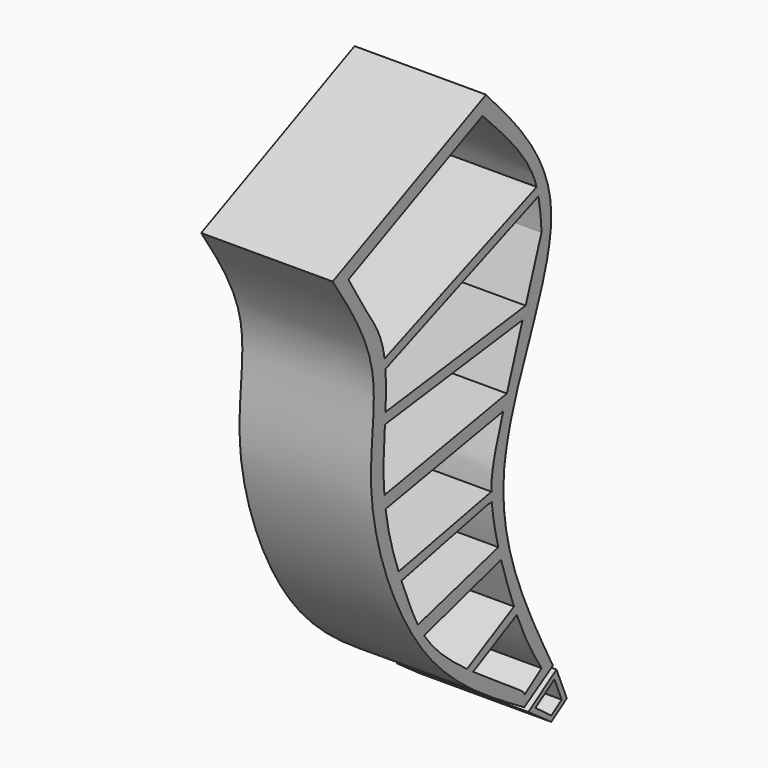
from build123d import *

# Parameters (mm, degrees)
F1_DEPTH  = 25
F2_DEPTH  = 25
F3_DEPTH  = 25
F4_DEPTH  = 25
F5_DEPTH  = 25
F6_DEPTH  = 25
F7_DEPTH  = 25
F10_DEPTH = 1
F11_DEPTH = 1


with BuildPart() as f1:
    # F0 (on Right) → F1 (new body)
    with BuildSketch(Plane.YZ):
        with BuildLine():
            Line((76.8012625446, 52.4432235212), (40.3474546597, 35.9775048702))
            add(Edge.make_bspline(
                [(40.3474546597, 35.9775048702), (44.5158897869, 29.6814892591), (52.7818571842, 17.1992282489), (46.5552937226, -3.8418948455), (59.8918941993, -37.9753033909), (77.3855119754, -48.6559954876), (85.8946596675, -53.8051620452)],
                knots=[0, 0, 0, 0, 0.225066194, 0.4463115245, 0.7316938963, 1, 1, 1, 1], degree=3))
            Line((85.8946596675, -53.8051620452), (92.699803412, -49.599211663))
            add(Edge.make_bspline(
                [(76.8012625446, 52.4432235212), (84.5131378217, 44.1641811003), (100.9174434445, 26.5534266137), (73.0582859494, -12.006269763), (86.1284394595, -37.021929702), (92.699803412, -49.599211663)],
                knots=[0, 0, 0, 0, 0.3061020156, 0.6511245107, 1, 1, 1, 1], degree=3))
        make_face()
        with BuildLine():
            add(Edge.make_bspline(
                [(44.102743268, 34.7667783499), (45.5869866773, 32.2564890577), (48.3654293439, 27.5573155976), (51.5365048206, 23.133247426), (52.4618114074, 19.5054126847), (52.6898807242, 18.0451917615)],
                knots=[0, 0, 0, 0, 0.1013554355, 0.1897091451, 0.2415289385, 0.2415289385, 0.2415289385, 0.2415289385], degree=3))
            Line((44.102743268, 34.7667783499), (75.9686642859, 49.2430719943))
            add(Edge.make_bspline(
                [(75.9686642859, 49.2430719943), (80.7651980081, 44.3752599295), (86.4678121426, 38.5879027477), (88.5720183844, 32.9802603832), (88.8379309187, 32.0926870872)],
                knots=[0, 0, 0, 0, 0.5664602164, 0.6734663454, 0.6734663454, 0.6734663454, 0.6734663454], degree=3))
            add(Edge.make_bspline(
                [(88.8379309187, 32.0926870872), (89.0099371396, 31.5185579706), (89.1533143996, 30.9458586664), (89.2741313424, 30.3742860892)],
                knots=[0.6734663454, 0.6734663454, 0.6734663454, 0.6734663454, 0.7426835409, 0.7426835409, 0.7426835409, 0.7426835409], degree=3))
            add(Edge.make_bspline(
                [(89.2741313424, 30.3742860892), (89.7232710063, 28.2494523594), (89.8606277376, 26.140189964), (89.9979844689, 24.0309275687)],
                knots=[0.7426835409, 0.7426835409, 0.7426835409, 0.7426835409, 1, 1, 1, 1], degree=3))
            add(Edge.make_bspline(
                [(89.9979844689, 24.0309275687), (88.756802073, 20.5110691156), (87.5156196771, 16.9912106625), (86.221231401, 13.2950814443)],
                knots=[0, 0, 0, 0, 0.1371374041, 0.1371374041, 0.1371374041, 0.1371374041], degree=3))
            add(Edge.make_bspline(
                [(86.221231401, 13.2950814443), (85.977143483, 12.5980877352), (85.7311635566, 11.8948258136), (85.4829348383, 11.1841136579)],
                knots=[0.1371374041, 0.1371374041, 0.1371374041, 0.1371374041, 0.162997947, 0.162997947, 0.162997947, 0.162997947], degree=3))
            add(Edge.make_bspline(
                [(85.4829348383, 11.1841136579), (85.267818915, 10.568207881), (84.035080256, 7.0343916925), (82.7402342637, 3.2948142782), (81.7634153644, 0.4019179056)],
                knots=[0.162997947, 0.162997947, 0.162997947, 0.162997947, 0.1854087888, 0.2904246225, 0.2904246225, 0.2904246225, 0.2904246225], degree=3))
            add(Edge.make_bspline(
                [(81.7634153644, 0.4019179056), (81.4591421255, -0.4992019947), (81.1636304992, -1.3819842427), (80.8808845893, -2.2364929875)],
                knots=[0.2904246225, 0.2904246225, 0.2904246225, 0.2904246225, 0.3231364259, 0.3231364259, 0.3231364259, 0.3231364259], degree=3))
            add(Edge.make_bspline(
                [(80.8808845893, -2.2364929875), (80.4400262019, -3.5688459381), (78.9176886377, -8.2626995613), (78.0330144779, -11.4884184754), (78.0771449208, -14.5385963842)],
                knots=[0.3231364259, 0.3231364259, 0.3231364259, 0.3231364259, 0.3741407815, 0.5125981189, 0.5125981189, 0.5125981189, 0.5125981189], degree=3))
            add(Edge.make_bspline(
                [(78.0771449208, -14.5385963842), (78.0854311956, -15.1113214854), (78.1180673371, -15.708474008), (78.1726109732, -16.3263524444)],
                knots=[0.5125981189, 0.5125981189, 0.5125981189, 0.5125981189, 0.5385959443, 0.5385959443, 0.5385959443, 0.5385959443], degree=3))
            add(Edge.make_bspline(
                [(78.1726109732, -16.3263524444), (78.3908448139, -18.7985379066), (78.9597891259, -21.6025182715), (79.7230046196, -24.5012038636)],
                knots=[0.5385959443, 0.5385959443, 0.5385959443, 0.5385959443, 0.6426155089, 0.6426155089, 0.6426155089, 0.6426155089], degree=3))
            add(Edge.make_bspline(
                [(79.7230046196, -24.5012038636), (79.9288007209, -25.2828156082), (80.1487218174, -26.0713131446), (80.3797008955, -26.8620482969)],
                knots=[0.6426155089, 0.6426155089, 0.6426155089, 0.6426155089, 0.6706637089, 0.6706637089, 0.6706637089, 0.6706637089], degree=3))
            add(Edge.make_bspline(
                [(80.3797008955, -26.8620482969), (80.5346897961, -27.3926382232), (81.4658723686, -30.4871004032), (82.53436506, -33.5681161087), (83.4502053618, -35.9443889597)],
                knots=[0.6706637089, 0.6706637089, 0.6706637089, 0.6706637089, 0.6894842867, 0.7802194818, 0.7802194818, 0.7802194818, 0.7802194818], degree=3))
            add(Edge.make_bspline(
                [(83.4502053618, -35.9443889597), (83.6683649907, -36.5104339378), (83.8882781867, -37.0665231191), (84.109089606, -37.61040963)],
                knots=[0.7802194818, 0.7802194818, 0.7802194818, 0.7802194818, 0.8018332462, 0.8018332462, 0.8018332462, 0.8018332462], degree=3))
            add(Edge.make_bspline(
                [(84.109089606, -37.61040963), (84.8138660141, -39.3463632453), (86.8646706616, -43.9759146648), (88.7614879392, -46.9768327841), (89.9979844689, -48.933070153)],
                knots=[0.8018332462, 0.8018332462, 0.8018332462, 0.8018332462, 0.8708191315, 1, 1, 1, 1], degree=3))
            add(Edge.make_bspline(
                [(89.9979844689, -48.933070153), (88.6734475692, -49.8509593308), (87.3239142246, -50.7842976763), (85.9993773248, -51.7021868541)],
                knots=[0, 0, 0, 0, 4.8638324804, 4.8638324804, 4.8638324804, 4.8638324804], degree=3))
            add(Edge.make_bspline(
                [(73.7536014428, -42.9259891452), (79.2616839922, -46.8631805496), (86.037278468, -51.0030413418), (85.9922818168, -51.6108465033), (85.9993773248, -51.7021868541)],
                knots=[0.8608913016, 0.8608913016, 0.8608913016, 0.8608913016, 0.9773228143, 1, 1, 1, 1], degree=3))
            add(Edge.make_bspline(
                [(72.2871573894, -41.8626360836), (72.7723382988, -42.2198965256), (73.2623216333, -42.5748210889), (73.7536014428, -42.9259891452)],
                knots=[0.8505064806, 0.8505064806, 0.8505064806, 0.8505064806, 0.8608913016, 0.8608913016, 0.8608913016, 0.8608913016], degree=3))
            add(Edge.make_bspline(
                [(62.0953731802, -32.1328573769), (63.2607762114, -33.8249216397), (65.9221012078, -36.948023318), (70.276587401, -40.3821633179), (72.2871573894, -41.8626360836)],
                knots=[0.7533164578, 0.7533164578, 0.7533164578, 0.7533164578, 0.807472204, 0.8505064806, 0.8505064806, 0.8505064806, 0.8505064806], degree=3))
            add(Edge.make_bspline(
                [(60.6140407616, -29.7249532229), (61.0500389658, -30.5200602261), (61.5361490607, -31.3209123912), (62.0953731802, -32.1328573769)],
                knots=[0.7273295685, 0.7273295685, 0.7273295685, 0.7273295685, 0.7533164578, 0.7533164578, 0.7533164578, 0.7533164578], degree=3))
            add(Edge.make_bspline(
                [(56.7143509479, -20.7657126474), (57.2022867526, -22.0176289299), (58.4314466262, -25.0352506359), (59.6503652252, -27.9675488107), (60.6140407616, -29.7249532229)],
                knots=[0.629936332, 0.629936332, 0.629936332, 0.629936332, 0.6698914204, 0.7273295685, 0.7273295685, 0.7273295685, 0.7273295685], degree=3))
            add(Edge.make_bspline(
                [(56.023799175, -18.9501089583), (56.2488718487, -19.5585059667), (56.479724527, -20.1637223163), (56.7143509479, -20.7657126474)],
                knots=[0.6107237239, 0.6107237239, 0.6107237239, 0.6107237239, 0.629936332, 0.629936332, 0.629936332, 0.629936332], degree=3))
            add(Edge.make_bspline(
                [(52.9298675724, -7.2175439477), (53.1930874664, -9.0898648938), (53.9905101976, -13.0627263871), (55.2720652308, -16.9180866991), (56.023799175, -18.9501089583)],
                knots=[0.4910644354, 0.4910644354, 0.4910644354, 0.4910644354, 0.5465543628, 0.6107237239, 0.6107237239, 0.6107237239, 0.6107237239], degree=3))
            add(Edge.make_bspline(
                [(52.6497218639, -4.78632948), (52.7232859651, -5.6025209503), (52.816732962, -6.4128011999), (52.9298675724, -7.2175439477)],
                knots=[0.4672142955, 0.4672142955, 0.4672142955, 0.4672142955, 0.4910644354, 0.4910644354, 0.4910644354, 0.4910644354], degree=3))
            add(Edge.make_bspline(
                [(52.7753754315, 6.992655232), (52.6218918281, 4.68010238), (52.3429405378, 0.660525646), (52.5079813052, -3.2137222818), (52.6497218639, -4.78632948)],
                knots=[0.3555619538, 0.3555619538, 0.3555619538, 0.3555619538, 0.4212607378, 0.4672142955, 0.4672142955, 0.4672142955, 0.4672142955], degree=3))
            add(Edge.make_bspline(
                [(52.9043617104, 9.0255401907), (52.8651208941, 8.3542760315), (52.8207131366, 7.6757629835), (52.7753754315, 6.992655232)],
                knots=[0.3361551115, 0.3361551115, 0.3361551115, 0.3361551115, 0.3555619538, 0.3555619538, 0.3555619538, 0.3555619538], degree=3))
            add(Edge.make_bspline(
                [(52.9090998165, 16.242469639), (52.9936284832, 15.2983602445), (53.0966265832, 12.9902209855), (52.9901220017, 10.4925792381), (52.9043617104, 9.0255401907)],
                knots=[0.2622006915, 0.2622006915, 0.2622006915, 0.2622006915, 0.2937417112, 0.3361551115, 0.3361551115, 0.3361551115, 0.3361551115], degree=3))
            add(Edge.make_bspline(
                [(52.6898807242, 18.0451917615), (52.7808612605, 17.4626860367), (52.8537003481, 16.8612320142), (52.9090998165, 16.242469639)],
                knots=[0.2415289385, 0.2415289385, 0.2415289385, 0.2415289385, 0.2622006915, 0.2622006915, 0.2622006915, 0.2622006915], degree=3))
        make_face(mode=Mode.SUBTRACT)
    extrude(amount=F1_DEPTH)

    # F0 (on Right) → F2 (join)
    with BuildSketch(Plane.YZ):
        with BuildLine():
            Line((88.8379309186, 32.0926870872), (52.6898807242, 18.0451917615))
            add(Edge.make_bspline(
                [(52.6898807242, 18.0451917615), (52.7808612605, 17.4626860367), (52.8537003481, 16.8612320142), (52.9090998165, 16.242469639)],
                knots=[0.2415289385, 0.2415289385, 0.2415289385, 0.2415289385, 0.2622006915, 0.2622006915, 0.2622006915, 0.2622006915], degree=3))
            Line((52.9090998165, 16.242469639), (89.2741313424, 30.3742860892))
            add(Edge.make_bspline(
                [(88.8379309187, 32.0926870872), (89.0099371396, 31.5185579706), (89.1533143996, 30.9458586664), (89.2741313424, 30.3742860892)],
                knots=[0.6734663454, 0.6734663454, 0.6734663454, 0.6734663454, 0.7426835409, 0.7426835409, 0.7426835409, 0.7426835409], degree=3))
        make_face()
    extrude(amount=F2_DEPTH)

    # F0 (on Right) → F3 (join)
    with BuildSketch(Plane.YZ):
        with BuildLine():
            Line((86.221231401, 13.2950814443), (52.9043617104, 9.0255401907))
            add(Edge.make_bspline(
                [(52.9043617104, 9.0255401907), (52.8651208941, 8.3542760315), (52.8207131366, 7.6757629835), (52.7753754315, 6.992655232)],
                knots=[0.3361551115, 0.3361551115, 0.3361551115, 0.3361551115, 0.3555619538, 0.3555619538, 0.3555619538, 0.3555619538], degree=3))
            Line((52.7753754315, 6.992655232), (85.4829348383, 11.1841136579))
            add(Edge.make_bspline(
                [(86.221231401, 13.2950814443), (85.977143483, 12.5980877352), (85.7311635566, 11.8948258136), (85.4829348383, 11.1841136579)],
                knots=[0.1371374041, 0.1371374041, 0.1371374041, 0.1371374041, 0.162997947, 0.162997947, 0.162997947, 0.162997947], degree=3))
        make_face()
    extrude(amount=F3_DEPTH)

    # F0 (on Right) → F4 (join)
    with BuildSketch(Plane.YZ):
        with BuildLine():
            Line((81.7634153644, 0.4019179056), (52.6497218639, -4.78632948))
            add(Edge.make_bspline(
                [(52.6497218639, -4.78632948), (52.7232859651, -5.6025209503), (52.816732962, -6.4128011999), (52.9298675724, -7.2175439477)],
                knots=[0.4672142955, 0.4672142955, 0.4672142955, 0.4672142955, 0.4910644354, 0.4910644354, 0.4910644354, 0.4910644354], degree=3))
            Line((52.9298675724, -7.2175439477), (80.8808845893, -2.2364929875))
            add(Edge.make_bspline(
                [(81.7634153644, 0.4019179056), (81.4591421255, -0.4992019947), (81.1636304992, -1.3819842427), (80.8808845893, -2.2364929875)],
                knots=[0.2904246225, 0.2904246225, 0.2904246225, 0.2904246225, 0.3231364259, 0.3231364259, 0.3231364259, 0.3231364259], degree=3))
        make_face()
    extrude(amount=F4_DEPTH)

    # F0 (on Right) → F5 (join)
    with BuildSketch(Plane.YZ):
        with BuildLine():
            Line((78.0771449208, -14.5385963842), (56.023799175, -18.9501089583))
            add(Edge.make_bspline(
                [(56.023799175, -18.9501089583), (56.2488718487, -19.5585059667), (56.479724527, -20.1637223163), (56.7143509479, -20.7657126474)],
                knots=[0.6107237239, 0.6107237239, 0.6107237239, 0.6107237239, 0.629936332, 0.629936332, 0.629936332, 0.629936332], degree=3))
            Line((56.7143509479, -20.7657126474), (77.2671707729, -16.3263524444))
            Line((77.2671707729, -16.3263524444), (78.1726109732, -16.3263524444))
            add(Edge.make_bspline(
                [(78.0771449208, -14.5385963842), (78.0854311956, -15.1113214854), (78.1180673371, -15.708474008), (78.1726109732, -16.3263524444)],
                knots=[0.5125981189, 0.5125981189, 0.5125981189, 0.5125981189, 0.5385959443, 0.5385959443, 0.5385959443, 0.5385959443], degree=3))
        make_face()
    extrude(amount=F5_DEPTH)

    # F0 (on Right) → F6 (join)
    with BuildSketch(Plane.YZ):
        with BuildLine():
            Line((79.7230046196, -24.5012038636), (60.6140407616, -29.7249532229))
            add(Edge.make_bspline(
                [(60.6140407616, -29.7249532229), (61.0500389658, -30.5200602261), (61.5361490607, -31.3209123912), (62.0953731802, -32.1328573769)],
                knots=[0.7273295685, 0.7273295685, 0.7273295685, 0.7273295685, 0.7533164578, 0.7533164578, 0.7533164578, 0.7533164578], degree=3))
            Line((62.0953731802, -32.1328573769), (80.3797008955, -26.8620482969))
            add(Edge.make_bspline(
                [(79.7230046196, -24.5012038636), (79.9288007209, -25.2828156082), (80.1487218174, -26.0713131446), (80.3797008955, -26.8620482969)],
                knots=[0.6426155089, 0.6426155089, 0.6426155089, 0.6426155089, 0.6706637089, 0.6706637089, 0.6706637089, 0.6706637089], degree=3))
        make_face()
    extrude(amount=F6_DEPTH)

    # F0 (on Right) → F7 (join)
    with BuildSketch(Plane.YZ):
        with BuildLine():
            Line((83.4502053618, -35.9443889597), (72.2871573894, -41.8626360836))
            add(Edge.make_bspline(
                [(72.2871573894, -41.8626360836), (72.7723382988, -42.2198965256), (73.2623216333, -42.5748210889), (73.7536014428, -42.9259891452)],
                knots=[0.8505064806, 0.8505064806, 0.8505064806, 0.8505064806, 0.8608913016, 0.8608913016, 0.8608913016, 0.8608913016], degree=3))
            Line((73.7536014428, -42.9259891452), (84.109089606, -37.61040963))
            add(Edge.make_bspline(
                [(83.4502053618, -35.9443889597), (83.6683649907, -36.5104339378), (83.8882781867, -37.0665231191), (84.109089606, -37.61040963)],
                knots=[0.7802194818, 0.7802194818, 0.7802194818, 0.7802194818, 0.8018332462, 0.8018332462, 0.8018332462, 0.8018332462], degree=3))
        make_face()
    extrude(amount=F7_DEPTH)


with BuildPart() as f1b:
    # F0 (on Right) → F1, piece 2 (new body)
    with BuildSketch(Plane.YZ):
        Polygon((93.5478610859, -50.5871062748), (86.8721157312, -54.9955554307), (92.3091694713, -58.8661059737), (96.0069314157, -56.4242220108), align=None)
        Polygon((92.3091694713, -57.8015310683), (88.5542035103, -54.9955554307), (93.0576155611, -52.0216458522), (94.7997059314, -56.156860283), align=None, mode=Mode.SUBTRACT)
    extrude(amount=F1_DEPTH)


with BuildPart() as f10:
    # F9 (on offset) → F10 (new body)
    with BuildSketch(Plane(origin=(0, 0, 0), x_dir=(0, -1, 0), z_dir=(-1, 0, 0))):
        with BuildLine():
            add(Edge.make_bspline(
                [(-75.9686642859, 49.2430719943), (-65.3466906133, 44.4176407795), (-54.7247169407, 39.5922095647), (-44.102743268, 34.7667783499)],
                knots=[0, 0, 0, 0, 35, 35, 35, 35], degree=3))
            add(Edge.make_bspline(
                [(-75.9686642859, 49.2430719943), (-78.66129457, 46.6755219245), (-83.9903281299, 41.5940368911), (-87.233469527, 35.2374474134), (-88.837930919, 32.0926870862)],
                knots=[0, 0, 0, 0, 0.5052755352, 1, 1, 1, 1], degree=3))
            add(Edge.make_bspline(
                [(-88.837930919, 32.0926870862), (-76.788580854, 27.4101886451), (-64.739230789, 22.7276902041), (-52.689880724, 18.0451917631)],
                knots=[0, 0, 0, 0, 38.7816149451, 38.7816149451, 38.7816149451, 38.7816149451], degree=3))
            add(Edge.make_bspline(
                [(-44.102743268, 34.7667783499), (-45.8580037651, 31.8560220837), (-48.8950957621, 26.8196078013), (-51.8328315201, 22.5455398579), (-52.4106929353, 19.5112090299), (-52.689880724, 18.0451917631)],
                knots=[0, 0, 0, 0, 0.4144400443, 0.7170897725, 1, 1, 1, 1], degree=3))
        make_face()
    extrude(amount=-F10_DEPTH)


with BuildPart() as f10b:
    # F9 (on offset) → F10, piece 2 (new body)
    with BuildSketch(Plane(origin=(0, 0, 0), x_dir=(0, -1, 0), z_dir=(-1, 0, 0))):
        with BuildLine():
            add(Edge.make_bspline(
                [(-89.2741313426, 30.3742860884), (-77.1524541671, 25.663680606), (-65.0307769917, 20.9530751235), (-52.9090998163, 16.2424696411)],
                knots=[0, 0, 0, 0, 39.0144044426, 39.0144044426, 39.0144044426, 39.0144044426], degree=3))
            add(Edge.make_bspline(
                [(-89.2741313426, 30.3742860884), (-89.8685955616, 28.5150743963), (-91.2921272563, 24.062919521), (-88.0875709088, 17.2581763669), (-86.2212314015, 13.2950814457)],
                knots=[0, 0, 0, 0, 0.4175981618, 1, 1, 1, 1], degree=3))
            add(Edge.make_bspline(
                [(-52.9043617106, 9.0255401932), (-64.0099849409, 10.4487206107), (-75.1156081712, 11.8719010282), (-86.2212314015, 13.2950814457)],
                knots=[0, 0, 0, 0, 33.5893255143, 33.5893255143, 33.5893255143, 33.5893255143], degree=3))
            add(Edge.make_bspline(
                [(-52.9090998163, 16.2424696411), (-52.9075204477, 13.8368264918), (-52.9059410791, 11.4311833425), (-52.9043617106, 9.0255401932)],
                knots=[0, 0, 0, 0, 7.2169310032, 7.2169310032, 7.2169310032, 7.2169310032], degree=3))
        make_face()
    extrude(amount=-F10_DEPTH)


with BuildPart() as f10c:
    # F9 (on offset) → F10, piece 3 (new body)
    with BuildSketch(Plane(origin=(0, 0, 0), x_dir=(0, -1, 0), z_dir=(-1, 0, 0))):
        with BuildLine():
            add(Edge.make_bspline(
                [(-85.4829348402, 11.1841136634), (-74.5804150374, 9.7869608546), (-63.6778952346, 8.3898080457), (-52.7753754318, 6.9926552369)],
                knots=[0, 0, 0, 0, 32.9750324669, 32.9750324669, 32.9750324669, 32.9750324669], degree=3))
            add(Edge.make_bspline(
                [(-85.4829348402, 11.1841136634), (-84.2430950149, 7.5900484108), (-83.0032551897, 3.9959831582), (-81.7634153644, 0.4019179056)],
                knots=[0, 0, 0, 0, 11.4057253382, 11.4057253382, 11.4057253382, 11.4057253382], degree=3))
            add(Edge.make_bspline(
                [(-52.6497218631, -4.7863294703), (-62.3542863635, -3.0569136783), (-72.058850864, -1.3274978864), (-81.7634153644, 0.4019179056)],
                knots=[0, 0, 0, 0, 29.5723698767, 29.5723698767, 29.5723698767, 29.5723698767], degree=3))
            add(Edge.make_bspline(
                [(-52.7753754318, 6.9926552369), (-52.629764464, 5.0302460442), (-52.3385765641, 1.1058863612), (-52.5460148456, -2.8224105807), (-52.6497218631, -4.7863294703)],
                knots=[0, 0, 0, 0, 0.500058443, 1, 1, 1, 1], degree=3))
        make_face()
    extrude(amount=-F10_DEPTH)


with BuildPart() as f10d:
    # F9 (on offset) → F10, piece 4 (new body)
    with BuildSketch(Plane(origin=(0, 0, 0), x_dir=(0, -1, 0), z_dir=(-1, 0, 0))):
        with BuildLine():
            add(Edge.make_bspline(
                [(-80.8808845893, -2.2364929876), (-71.5638789166, -3.8968433045), (-62.2468732438, -5.5571936213), (-52.9298675711, -7.2175439382)],
                knots=[0, 0, 0, 0, 28.3913758196, 28.3913758196, 28.3913758196, 28.3913758196], degree=3))
            add(Edge.make_bspline(
                [(-80.8808845893, -2.2364929876), (-80.1631109469, -4.2347182609), (-78.7288687651, -8.2275378818), (-78.2942557626, -12.4361863007), (-78.0771449208, -14.5385963842)],
                knots=[0, 0, 0, 0, 0.5004567325, 1, 1, 1, 1], degree=3))
            Line((-78.0771449208, -14.5385963842), (-56.0237991752, -19.1139187664))
            add(Edge.make_bspline(
                [(-52.9298675711, -7.2175439382), (-53.2836007921, -9.2084246591), (-53.9956375963, -13.2158988545), (-55.3448600225, -17.1395203588), (-56.0237991752, -19.1139187664)],
                knots=[0, 0, 0, 0, 0.496793811, 1, 1, 1, 1], degree=3))
        make_face()
    extrude(amount=-F10_DEPTH)


with BuildPart() as f10e:
    # F9 (on offset) → F10, piece 5 (new body)
    with BuildSketch(Plane(origin=(0, 0, 0), x_dir=(0, -1, 0), z_dir=(-1, 0, 0))):
        with BuildLine():
            add(Edge.make_bspline(
                [(-78.1726109732, -16.3263524444), (-71.0198576318, -17.8061391798), (-63.8671042904, -19.2859259151), (-56.7143509491, -20.7657126505)],
                knots=[0, 0, 0, 0, 21.9126639709, 21.9126639709, 21.9126639709, 21.9126639709], degree=3))
            add(Edge.make_bspline(
                [(-78.1726109732, -16.3263524444), (-78.6894088551, -19.0513029165), (-79.206206737, -21.7762533885), (-79.7230046188, -24.5012038606)],
                knots=[0, 0, 0, 0, 8.3205718633, 8.3205718633, 8.3205718633, 8.3205718633], degree=3))
            add(Edge.make_bspline(
                [(-79.7230046188, -24.5012038606), (-73.3533499988, -26.2424536463), (-66.9836953787, -27.9837034319), (-60.6140407587, -29.7249532176)],
                knots=[0, 0, 0, 0, 19.8100998774, 19.8100998774, 19.8100998774, 19.8100998774], degree=3))
            add(Edge.make_bspline(
                [(-60.6140407587, -29.7249532176), (-59.9249396818, -28.2492285732), (-59.2358386049, -26.7735039289), (-58.546737528, -25.2977792845)],
                knots=[0, 0, 0, 0, 4.8860630042, 4.8860630042, 4.8860630042, 4.8860630042], degree=3))
            add(Edge.make_bspline(
                [(-56.7143509491, -20.7657126505), (-57.3251464754, -22.2764015285), (-57.9359420017, -23.7870904065), (-58.546737528, -25.2977792845)],
                knots=[0, 0, 0, 0, 4.8884832566, 4.8884832566, 4.8884832566, 4.8884832566], degree=3))
        make_face()
    extrude(amount=-F10_DEPTH)


with BuildPart() as f10f:
    # F9 (on offset) → F10, piece 6 (new body)
    with BuildSketch(Plane(origin=(0, 0, 0), x_dir=(0, -1, 0), z_dir=(-1, 0, 0))):
        with BuildLine():
            add(Edge.make_bspline(
                [(-80.3797008953, -26.8620482963), (-74.2849249903, -28.6189846565), (-68.1901490852, -30.3759210167), (-62.0953731802, -32.1328573769)],
                knots=[0, 0, 0, 0, 19.0288745951, 19.0288745951, 19.0288745951, 19.0288745951], degree=3))
            add(Edge.make_bspline(
                [(-80.3797008953, -26.8620482963), (-81.4032023841, -29.8894951841), (-82.4267038729, -32.9169420719), (-83.4502053618, -35.9443889597)],
                knots=[0, 0, 0, 0, 9.587330682, 9.587330682, 9.587330682, 9.587330682], degree=3))
            add(Edge.make_bspline(
                [(-83.4502053618, -35.9443889597), (-79.7291893699, -37.9171380002), (-76.008173378, -39.8898870407), (-72.2871573862, -41.8626360812)],
                knots=[0, 0, 0, 0, 12.634844245, 12.634844245, 12.634844245, 12.634844245], degree=3))
            add(Edge.make_bspline(
                [(-72.2871573862, -41.8626360812), (-70.3832200798, -40.451501737), (-66.5690945636, -37.6419432497), (-63.5887960988, -33.9648805667), (-62.0953731802, -32.1328573769)],
                knots=[0, 0, 0, 0, 0.5002195831, 1, 1, 1, 1], degree=3))
        make_face()
    extrude(amount=-F10_DEPTH)


with BuildPart() as f10g:
    # F9 (on offset) → F10, piece 7 (new body)
    with BuildSketch(Plane(origin=(0, 0, 0), x_dir=(0, -1, 0), z_dir=(-1, 0, 0))):
        with BuildLine():
            add(Edge.make_bspline(
                [(-84.109089606, -37.61040963), (-80.6572602153, -39.3822694663), (-77.2054308246, -41.1541293026), (-73.7536014339, -42.9259891389)],
                knots=[0, 0, 0, 0, 11.6400825082, 11.6400825082, 11.6400825082, 11.6400825082], degree=3))
            add(Edge.make_bspline(
                [(-84.109089606, -37.61040963), (-84.9914253862, -39.5490575861), (-85.8737921147, -41.4877650511), (-86.756127895, -43.4264130072)],
                knots=[0, 0, 0, 0, 6.3900474949, 6.3900474949, 6.3900474949, 6.3900474949], degree=3))
            add(Edge.make_bspline(
                [(-89.9979844689, -48.933070153), (-88.9173552948, -47.0974979348), (-87.836757069, -45.2619852254), (-86.756127895, -43.4264130072)],
                knots=[0, 0, 0, 0, 6.3900631427, 6.3900631427, 6.3900631427, 6.3900631427], degree=3))
            add(Edge.make_bspline(
                [(-89.9979844689, -48.933070153), (-88.6651154209, -49.8561090534), (-87.3322463729, -50.7791479537), (-85.9993773248, -51.7021868541)],
                knots=[0, 0, 0, 0, 4.8638324804, 4.8638324804, 4.8638324804, 4.8638324804], degree=3))
            add(Edge.make_bspline(
                [(-73.7536014339, -42.9259891389), (-77.8355267309, -45.8513883773), (-81.9174520279, -48.7767876157), (-85.9993773248, -51.7021868541)],
                knots=[0, 0, 0, 0, 15.0658777875, 15.0658777875, 15.0658777875, 15.0658777875], degree=3))
        make_face()
    extrude(amount=-F10_DEPTH)


with BuildPart() as f10h:
    # F9 (on offset) → F10, piece 8 (new body)
    with BuildSketch(Plane(origin=(0, 0, 0), x_dir=(0, -1, 0), z_dir=(-1, 0, 0))):
        with BuildLine():
            add(Edge.make_bspline(
                [(-93.0576155611, -52.0216458522), (-91.5564782108, -53.012949045), (-90.0553408606, -54.0042522378), (-88.5542035103, -54.9955554307)],
                knots=[0, 0, 0, 0, 5.3967451562, 5.3967451562, 5.3967451562, 5.3967451562], degree=3))
            add(Edge.make_bspline(
                [(-94.7997059314, -56.156860283), (-94.2190091413, -54.7784554727), (-93.6383123512, -53.4000506624), (-93.0576155611, -52.0216458522)],
                knots=[0, 0, 0, 0, 4.4871903511, 4.4871903511, 4.4871903511, 4.4871903511], degree=3))
            add(Edge.make_bspline(
                [(-92.3091694713, -57.8015310683), (-93.1393482913, -57.2533074732), (-93.9695271114, -56.7050838781), (-94.7997059314, -56.156860283)],
                knots=[0, 0, 0, 0, 2.9845793425, 2.9845793425, 2.9845793425, 2.9845793425], degree=3))
            add(Edge.make_bspline(
                [(-88.5542035103, -54.9955554307), (-89.8058588306, -55.9308806432), (-91.0575141509, -56.8662058558), (-92.3091694713, -57.8015310683)],
                knots=[0, 0, 0, 0, 4.6875653219, 4.6875653219, 4.6875653219, 4.6875653219], degree=3))
        make_face()
    extrude(amount=-F10_DEPTH)


with BuildPart() as f11:
    # F9 (on offset) → F11 (new body)
    with BuildSketch(Plane(origin=(0, 0, 0), x_dir=(0, -1, 0), z_dir=(-1, 0, 0))):
        with BuildLine():
            add(Edge.make_bspline(
                [(-75.9686642859, 49.2430719943), (-65.3466906133, 44.4176407795), (-54.7247169407, 39.5922095647), (-44.102743268, 34.7667783499)],
                knots=[0, 0, 0, 0, 35, 35, 35, 35], degree=3))
            add(Edge.make_bspline(
                [(-75.9686642859, 49.2430719943), (-78.66129457, 46.6755219245), (-83.9903281299, 41.5940368911), (-87.233469527, 35.2374474134), (-88.837930919, 32.0926870862)],
                knots=[0, 0, 0, 0, 0.5052755352, 1, 1, 1, 1], degree=3))
            add(Edge.make_bspline(
                [(-88.837930919, 32.0926870862), (-76.788580854, 27.4101886451), (-64.739230789, 22.7276902041), (-52.689880724, 18.0451917631)],
                knots=[0, 0, 0, 0, 38.7816149451, 38.7816149451, 38.7816149451, 38.7816149451], degree=3))
            add(Edge.make_bspline(
                [(-44.102743268, 34.7667783499), (-45.8580037651, 31.8560220837), (-48.8950957621, 26.8196078013), (-51.8328315201, 22.5455398579), (-52.4106929353, 19.5112090299), (-52.689880724, 18.0451917631)],
                knots=[0, 0, 0, 0, 0.4144400443, 0.7170897725, 1, 1, 1, 1], degree=3))
        make_face()
    extrude(amount=-F11_DEPTH)


with BuildPart() as f11b:
    # F9 (on offset) → F11, piece 2 (new body)
    with BuildSketch(Plane(origin=(0, 0, 0), x_dir=(0, -1, 0), z_dir=(-1, 0, 0))):
        with BuildLine():
            add(Edge.make_bspline(
                [(-89.2741313426, 30.3742860884), (-77.1524541671, 25.663680606), (-65.0307769917, 20.9530751235), (-52.9090998163, 16.2424696411)],
                knots=[0, 0, 0, 0, 39.0144044426, 39.0144044426, 39.0144044426, 39.0144044426], degree=3))
            add(Edge.make_bspline(
                [(-89.2741313426, 30.3742860884), (-89.8685955616, 28.5150743963), (-91.2921272563, 24.062919521), (-88.0875709088, 17.2581763669), (-86.2212314015, 13.2950814457)],
                knots=[0, 0, 0, 0, 0.4175981618, 1, 1, 1, 1], degree=3))
            add(Edge.make_bspline(
                [(-52.9043617106, 9.0255401932), (-64.0099849409, 10.4487206107), (-75.1156081712, 11.8719010282), (-86.2212314015, 13.2950814457)],
                knots=[0, 0, 0, 0, 33.5893255143, 33.5893255143, 33.5893255143, 33.5893255143], degree=3))
            add(Edge.make_bspline(
                [(-52.9090998163, 16.2424696411), (-52.9075204477, 13.8368264918), (-52.9059410791, 11.4311833425), (-52.9043617106, 9.0255401932)],
                knots=[0, 0, 0, 0, 7.2169310032, 7.2169310032, 7.2169310032, 7.2169310032], degree=3))
        make_face()
    extrude(amount=-F11_DEPTH)


with BuildPart() as f11c:
    # F9 (on offset) → F11, piece 3 (new body)
    with BuildSketch(Plane(origin=(0, 0, 0), x_dir=(0, -1, 0), z_dir=(-1, 0, 0))):
        with BuildLine():
            add(Edge.make_bspline(
                [(-85.4829348402, 11.1841136634), (-74.5804150374, 9.7869608546), (-63.6778952346, 8.3898080457), (-52.7753754318, 6.9926552369)],
                knots=[0, 0, 0, 0, 32.9750324669, 32.9750324669, 32.9750324669, 32.9750324669], degree=3))
            add(Edge.make_bspline(
                [(-85.4829348402, 11.1841136634), (-84.2430950149, 7.5900484108), (-83.0032551897, 3.9959831582), (-81.7634153644, 0.4019179056)],
                knots=[0, 0, 0, 0, 11.4057253382, 11.4057253382, 11.4057253382, 11.4057253382], degree=3))
            add(Edge.make_bspline(
                [(-52.6497218631, -4.7863294703), (-62.3542863635, -3.0569136783), (-72.058850864, -1.3274978864), (-81.7634153644, 0.4019179056)],
                knots=[0, 0, 0, 0, 29.5723698767, 29.5723698767, 29.5723698767, 29.5723698767], degree=3))
            add(Edge.make_bspline(
                [(-52.7753754318, 6.9926552369), (-52.629764464, 5.0302460442), (-52.3385765641, 1.1058863612), (-52.5460148456, -2.8224105807), (-52.6497218631, -4.7863294703)],
                knots=[0, 0, 0, 0, 0.500058443, 1, 1, 1, 1], degree=3))
        make_face()
    extrude(amount=-F11_DEPTH)


with BuildPart() as f11d:
    # F9 (on offset) → F11, piece 4 (new body)
    with BuildSketch(Plane(origin=(0, 0, 0), x_dir=(0, -1, 0), z_dir=(-1, 0, 0))):
        with BuildLine():
            add(Edge.make_bspline(
                [(-80.8808845893, -2.2364929876), (-71.5638789166, -3.8968433045), (-62.2468732438, -5.5571936213), (-52.9298675711, -7.2175439382)],
                knots=[0, 0, 0, 0, 28.3913758196, 28.3913758196, 28.3913758196, 28.3913758196], degree=3))
            add(Edge.make_bspline(
                [(-80.8808845893, -2.2364929876), (-80.1631109469, -4.2347182609), (-78.7288687651, -8.2275378818), (-78.2942557626, -12.4361863007), (-78.0771449208, -14.5385963842)],
                knots=[0, 0, 0, 0, 0.5004567325, 1, 1, 1, 1], degree=3))
            Line((-78.0771449208, -14.5385963842), (-56.0237991752, -19.1139187664))
            add(Edge.make_bspline(
                [(-52.9298675711, -7.2175439382), (-53.2836007921, -9.2084246591), (-53.9956375963, -13.2158988545), (-55.3448600225, -17.1395203588), (-56.0237991752, -19.1139187664)],
                knots=[0, 0, 0, 0, 0.496793811, 1, 1, 1, 1], degree=3))
        make_face()
    extrude(amount=-F11_DEPTH)


with BuildPart() as f11e:
    # F9 (on offset) → F11, piece 5 (new body)
    with BuildSketch(Plane(origin=(0, 0, 0), x_dir=(0, -1, 0), z_dir=(-1, 0, 0))):
        with BuildLine():
            add(Edge.make_bspline(
                [(-78.1726109732, -16.3263524444), (-71.0198576318, -17.8061391798), (-63.8671042904, -19.2859259151), (-56.7143509491, -20.7657126505)],
                knots=[0, 0, 0, 0, 21.9126639709, 21.9126639709, 21.9126639709, 21.9126639709], degree=3))
            add(Edge.make_bspline(
                [(-78.1726109732, -16.3263524444), (-78.6894088551, -19.0513029165), (-79.206206737, -21.7762533885), (-79.7230046188, -24.5012038606)],
                knots=[0, 0, 0, 0, 8.3205718633, 8.3205718633, 8.3205718633, 8.3205718633], degree=3))
            add(Edge.make_bspline(
                [(-79.7230046188, -24.5012038606), (-73.3533499988, -26.2424536463), (-66.9836953787, -27.9837034319), (-60.6140407587, -29.7249532176)],
                knots=[0, 0, 0, 0, 19.8100998774, 19.8100998774, 19.8100998774, 19.8100998774], degree=3))
            add(Edge.make_bspline(
                [(-60.6140407587, -29.7249532176), (-59.9249396818, -28.2492285732), (-59.2358386049, -26.7735039289), (-58.546737528, -25.2977792845)],
                knots=[0, 0, 0, 0, 4.8860630042, 4.8860630042, 4.8860630042, 4.8860630042], degree=3))
            add(Edge.make_bspline(
                [(-56.7143509491, -20.7657126505), (-57.3251464754, -22.2764015285), (-57.9359420017, -23.7870904065), (-58.546737528, -25.2977792845)],
                knots=[0, 0, 0, 0, 4.8884832566, 4.8884832566, 4.8884832566, 4.8884832566], degree=3))
        make_face()
    extrude(amount=-F11_DEPTH)


with BuildPart() as f11f:
    # F9 (on offset) → F11, piece 6 (new body)
    with BuildSketch(Plane(origin=(0, 0, 0), x_dir=(0, -1, 0), z_dir=(-1, 0, 0))):
        with BuildLine():
            add(Edge.make_bspline(
                [(-80.3797008953, -26.8620482963), (-74.2849249903, -28.6189846565), (-68.1901490852, -30.3759210167), (-62.0953731802, -32.1328573769)],
                knots=[0, 0, 0, 0, 19.0288745951, 19.0288745951, 19.0288745951, 19.0288745951], degree=3))
            add(Edge.make_bspline(
                [(-80.3797008953, -26.8620482963), (-81.4032023841, -29.8894951841), (-82.4267038729, -32.9169420719), (-83.4502053618, -35.9443889597)],
                knots=[0, 0, 0, 0, 9.587330682, 9.587330682, 9.587330682, 9.587330682], degree=3))
            add(Edge.make_bspline(
                [(-83.4502053618, -35.9443889597), (-79.7291893699, -37.9171380002), (-76.008173378, -39.8898870407), (-72.2871573862, -41.8626360812)],
                knots=[0, 0, 0, 0, 12.634844245, 12.634844245, 12.634844245, 12.634844245], degree=3))
            add(Edge.make_bspline(
                [(-72.2871573862, -41.8626360812), (-70.3832200798, -40.451501737), (-66.5690945636, -37.6419432497), (-63.5887960988, -33.9648805667), (-62.0953731802, -32.1328573769)],
                knots=[0, 0, 0, 0, 0.5002195831, 1, 1, 1, 1], degree=3))
        make_face()
    extrude(amount=-F11_DEPTH)


with BuildPart() as f11g:
    # F9 (on offset) → F11, piece 7 (new body)
    with BuildSketch(Plane(origin=(0, 0, 0), x_dir=(0, -1, 0), z_dir=(-1, 0, 0))):
        with BuildLine():
            add(Edge.make_bspline(
                [(-84.109089606, -37.61040963), (-80.6572602153, -39.3822694663), (-77.2054308246, -41.1541293026), (-73.7536014339, -42.9259891389)],
                knots=[0, 0, 0, 0, 11.6400825082, 11.6400825082, 11.6400825082, 11.6400825082], degree=3))
            add(Edge.make_bspline(
                [(-84.109089606, -37.61040963), (-84.9914253862, -39.5490575861), (-85.8737921147, -41.4877650511), (-86.756127895, -43.4264130072)],
                knots=[0, 0, 0, 0, 6.3900474949, 6.3900474949, 6.3900474949, 6.3900474949], degree=3))
            add(Edge.make_bspline(
                [(-89.9979844689, -48.933070153), (-88.9173552948, -47.0974979348), (-87.836757069, -45.2619852254), (-86.756127895, -43.4264130072)],
                knots=[0, 0, 0, 0, 6.3900631427, 6.3900631427, 6.3900631427, 6.3900631427], degree=3))
            add(Edge.make_bspline(
                [(-89.9979844689, -48.933070153), (-88.6651154209, -49.8561090534), (-87.3322463729, -50.7791479537), (-85.9993773248, -51.7021868541)],
                knots=[0, 0, 0, 0, 4.8638324804, 4.8638324804, 4.8638324804, 4.8638324804], degree=3))
            add(Edge.make_bspline(
                [(-73.7536014339, -42.9259891389), (-77.8355267309, -45.8513883773), (-81.9174520279, -48.7767876157), (-85.9993773248, -51.7021868541)],
                knots=[0, 0, 0, 0, 15.0658777875, 15.0658777875, 15.0658777875, 15.0658777875], degree=3))
        make_face()
    extrude(amount=-F11_DEPTH)


with BuildPart() as f11h:
    # F9 (on offset) → F11, piece 8 (new body)
    with BuildSketch(Plane(origin=(0, 0, 0), x_dir=(0, -1, 0), z_dir=(-1, 0, 0))):
        with BuildLine():
            add(Edge.make_bspline(
                [(-93.0576155611, -52.0216458522), (-91.5564782108, -53.012949045), (-90.0553408606, -54.0042522378), (-88.5542035103, -54.9955554307)],
                knots=[0, 0, 0, 0, 5.3967451562, 5.3967451562, 5.3967451562, 5.3967451562], degree=3))
            add(Edge.make_bspline(
                [(-94.7997059314, -56.156860283), (-94.2190091413, -54.7784554727), (-93.6383123512, -53.4000506624), (-93.0576155611, -52.0216458522)],
                knots=[0, 0, 0, 0, 4.4871903511, 4.4871903511, 4.4871903511, 4.4871903511], degree=3))
            add(Edge.make_bspline(
                [(-92.3091694713, -57.8015310683), (-93.1393482913, -57.2533074732), (-93.9695271114, -56.7050838781), (-94.7997059314, -56.156860283)],
                knots=[0, 0, 0, 0, 2.9845793425, 2.9845793425, 2.9845793425, 2.9845793425], degree=3))
            add(Edge.make_bspline(
                [(-88.5542035103, -54.9955554307), (-89.8058588306, -55.9308806432), (-91.0575141509, -56.8662058558), (-92.3091694713, -57.8015310683)],
                knots=[0, 0, 0, 0, 4.6875653219, 4.6875653219, 4.6875653219, 4.6875653219], degree=3))
        make_face()
    extrude(amount=-F11_DEPTH)


solid = Compound([f1.part, f1b.part, f10.part, f10b.part, f10c.part, f10d.part, f10e.part, f10f.part, f10g.part, f10h.part, f11.part, f11b.part, f11c.part, f11d.part, f11e.part, f11f.part, f11g.part, f11h.part])
